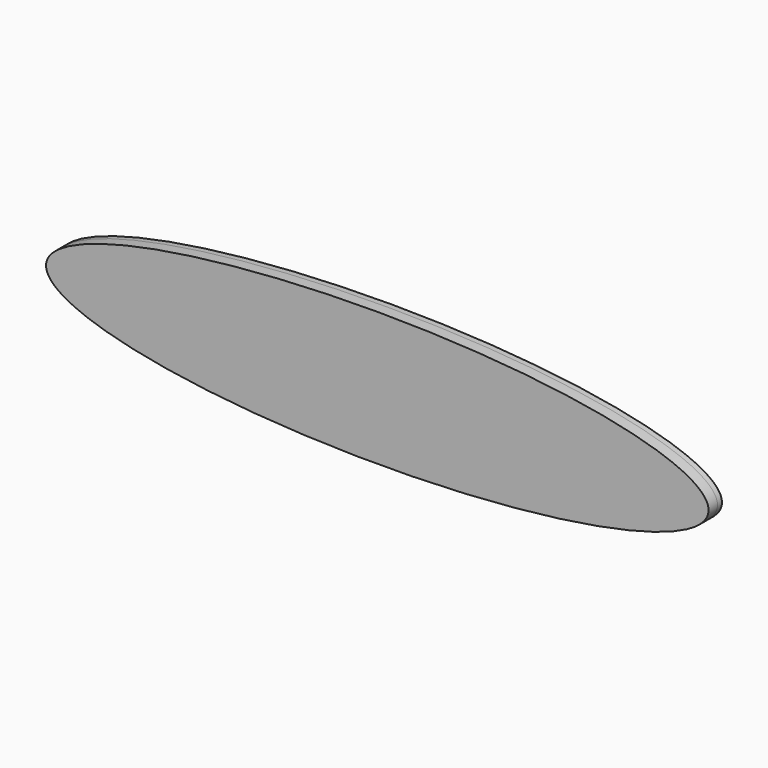
from build123d import *

# Parameters (mm, degrees)
F1_DEPTH = 1.5
F3_DEPTH = 3


# Not quite as in the source:
# - a feature names something its author has since deleted; it is built from what else it names


with BuildPart() as f1:
    # F0 (on Front) → F1 (new body)
    with BuildSketch(Plane.XZ):
        with BuildLine():
            add(Edge.make_bspline(
                [(-30.1864057183, 0), (-30.1864057183, -31.1769145362), (103.3135942817, -15.5884572681), (236.8135942817, 0), (103.3135942817, 15.5884572681), (-30.1864057183, 31.1769145362), (-30.1864057183, 0)],
                knots=[0, 0, 0, 2.0943951024, 2.0943951024, 4.1887902048, 4.1887902048, 6.2831853072, 6.2831853072, 6.2831853072], degree=2, weights=[1, 0.5, 1, 0.5, 1, 0.5, 1]))
        make_face()
    extrude(amount=F1_DEPTH)

    # F3 (add): a face of the model
    f3_faces = [f1.faces().sort_by_distance(p)[0] for p in [
        (58.705611849, -1.5, 0),
    ]]
    extrude(f3_faces, amount=F3_DEPTH)


solid = f1.part
